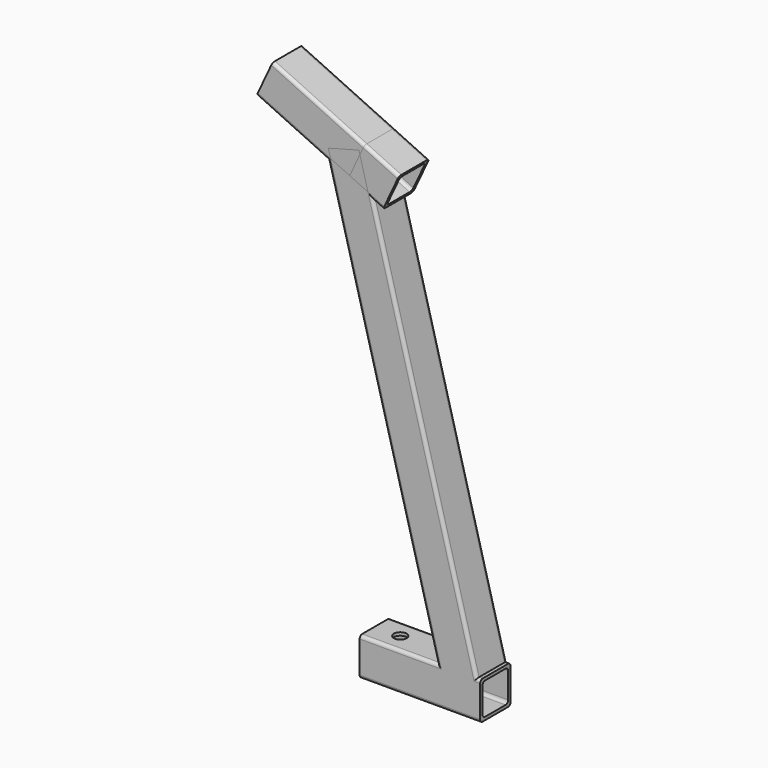
from build123d import *
from build123d import SkipClean  # not in build123d's __all__

# Parameters (mm, degrees)
F1_DEPTH       = 44.45
F1_DEPTH_BACK  = 76.2
F5_DEPTH       = 419.1
F5_DEPTH_BACK  = 28.956
F7_DEPTH       = 145.288
F10_DEPTH      = 38.1
F10_DEPTH_BACK = 101.6
F12_DEPTH      = 154.2941466414
F13_R          = 6.35
F14_DEPTH      = 6.35
F15_R          = 6.35
F16_DEPTH      = 6.35


with BuildPart() as f1:
    # F0 (on Right) → F1 (new body, two sides)
    with BuildSketch(Plane.YZ) as f1_sk:
        with BuildLine():
            ThreePointArc((19.05, 15.875), (18.1200640303, 18.1200640303), (15.875, 19.05))
            Line((15.875, 19.05), (-15.875, 19.05))
            ThreePointArc((-15.875, 19.05), (-18.1200640303, 18.1200640303), (-19.05, 15.875))
            Line((-19.05, 15.875), (-19.05, -15.875))
            ThreePointArc((-19.05, -15.875), (-18.1200640303, -18.1200640303), (-15.875, -19.05))
            Line((-15.875, -19.05), (15.875, -19.05))
            ThreePointArc((15.875, -19.05), (18.1200640303, -18.1200640303), (19.05, -15.875))
            Line((19.05, -15.875), (19.05, 15.875))
        make_face()
        with BuildLine():
            Line((-16.002, -12.827), (-16.002, 12.827))
            ThreePointArc((-16.002, 12.827), (-15.0720640303, 15.0720640303), (-12.827, 16.002))
            Line((-12.827, 16.002), (12.827, 16.002))
            ThreePointArc((12.827, 16.002), (15.0720640303, 15.0720640303), (16.002, 12.827))
            Line((16.002, 12.827), (16.002, -12.827))
            ThreePointArc((16.002, -12.827), (15.0720640303, -15.0720640303), (12.827, -16.002))
            Line((12.827, -16.002), (-12.827, -16.002))
            ThreePointArc((-12.827, -16.002), (-15.0720640303, -15.0720640303), (-16.002, -12.827))
        make_face(mode=Mode.SUBTRACT)
    extrude(amount=F1_DEPTH)
    extrude(f1_sk.sketch, amount=-F1_DEPTH_BACK)

    # F4 (on face) → F5 (join, two sides)
    with BuildSketch(Plane(origin=(-8.3589183447, 0, 31.1959079588), x_dir=(0.9659258263, 0, 0.2588190451), z_dir=(0.2588190451, 0, -0.9659258263))) as f5_sk:
        with BuildLine():
            ThreePointArc((44.45, 15.875), (43.5200640303, 18.1200640303), (41.275, 19.05))
            Line((41.275, 19.05), (9.525, 19.05))
            ThreePointArc((9.525, 19.05), (7.2799359697, 18.1200640303), (6.35, 15.875))
            Line((6.35, 15.875), (6.35, -15.875))
            ThreePointArc((6.35, -15.875), (7.2799359697, -18.1200640303), (9.525, -19.05))
            Line((9.525, -19.05), (41.275, -19.05))
            ThreePointArc((41.275, -19.05), (43.5200640303, -18.1200640303), (44.45, -15.875))
            Line((44.45, -15.875), (44.45, 15.875))
        make_face()
        with BuildLine():
            Line((12.573, 16.002), (38.227, 16.002))
            ThreePointArc((38.227, 16.002), (40.4720640303, 15.0720640303), (41.402, 12.827))
            Line((41.402, 12.827), (41.402, -12.827))
            ThreePointArc((41.402, -12.827), (40.4720640303, -15.0720640303), (38.227, -16.002))
            Line((38.227, -16.002), (12.573, -16.002))
            ThreePointArc((12.573, -16.002), (10.3279359697, -15.0720640303), (9.398, -12.827))
            Line((9.398, -12.827), (9.398, 12.827))
            ThreePointArc((9.398, 12.827), (10.3279359697, 15.0720640303), (12.573, 16.002))
        make_face(mode=Mode.SUBTRACT)
    extrude(amount=-F5_DEPTH)
    extrude(f5_sk.sketch, amount=F5_DEPTH_BACK)

    # F6 (on face) → F7 (cut)
    with BuildSketch(Plane(origin=(-76.2, 0, 0), x_dir=(0, -1, 0), z_dir=(-1, 0, 0))):
        with BuildLine():
            Line((12.827, 16.002), (-12.827, 16.002))
            ThreePointArc((-12.827, 16.002), (-15.0720640303, 15.0720640303), (-16.002, 12.827))
            Line((-16.002, 12.827), (-16.002, -12.827))
            ThreePointArc((-16.002, -12.827), (-15.0720640303, -15.0720640303), (-12.827, -16.002))
            Line((-12.827, -16.002), (12.827, -16.002))
            ThreePointArc((12.827, -16.002), (15.0720640303, -15.0720640303), (16.002, -12.827))
            Line((16.002, -12.827), (16.002, 12.827))
            ThreePointArc((16.002, 12.827), (15.0720640303, 15.0720640303), (12.827, 16.002))
        make_face()
    with SkipClean():  # cleaning this boolean's faces spoils the solid; the shape is the same uncleaned
        extrude(amount=-F7_DEPTH, mode=Mode.SUBTRACT)

    # F9 (on face) → F10 (join, two sides)
    with BuildSketch(Plane(origin=(-232.1066250318, 0, 108.2330967608), x_dir=(0, 1, 0), z_dir=(0.906307787, 0, -0.4226182617))) as f10_sk:
        with BuildLine():
            ThreePointArc((19.05, 377.0523048448), (18.1200640303, 379.297368875), (15.875, 380.2273048448))
            Line((15.875, 380.2273048448), (-15.875, 380.2273048448))
            ThreePointArc((-15.875, 380.2273048448), (-18.1200640303, 379.297368875), (-19.05, 377.0523048448))
            Line((-19.05, 377.0523048448), (-19.05, 345.3023048448))
            ThreePointArc((-19.05, 345.3023048448), (-18.1200640303, 343.0572408145), (-15.875, 342.1273048448))
            Line((-15.875, 342.1273048448), (15.875, 342.1273048448))
            ThreePointArc((15.875, 342.1273048448), (18.1200640303, 343.0572408145), (19.05, 345.3023048448))
            Line((19.05, 345.3023048448), (19.05, 377.0523048448))
        make_face()
        with BuildLine():
            Line((-12.827, 377.1793048448), (12.827, 377.1793048448))
            ThreePointArc((12.827, 377.1793048448), (15.0720640303, 376.249368875), (16.002, 374.0043048448))
            Line((16.002, 374.0043048448), (16.002, 348.3503048448))
            ThreePointArc((16.002, 348.3503048448), (15.0720640303, 346.1052408145), (12.827, 345.1753048448))
            Line((12.827, 345.1753048448), (-12.827, 345.1753048448))
            ThreePointArc((-12.827, 345.1753048448), (-15.0720640303, 346.1052408145), (-16.002, 348.3503048448))
            Line((-16.002, 348.3503048448), (-16.002, 374.0043048448))
            ThreePointArc((-16.002, 374.0043048448), (-15.0720640303, 376.249368875), (-12.827, 377.1793048448))
        make_face(mode=Mode.SUBTRACT)
    with SkipClean():  # cleaning this boolean's faces spoils the solid; the shape is the same uncleaned
        extrude(amount=F10_DEPTH)
        extrude(f10_sk.sketch, amount=-F10_DEPTH_BACK)

    # F11 (on face) → F12 (cut, through all)
    with BuildSketch(Plane(origin=(-197.5762983457, 0, 92.1313409885), x_dir=(0, 1, 0), z_dir=(0.906307787, 0, -0.4226182617))):
        with BuildLine():
            ThreePointArc((-12.827, 377.1793048448), (-15.0720640303, 376.249368875), (-16.002, 374.0043048448))
            Line((-16.002, 374.0043048448), (-16.002, 348.3503048448))
            ThreePointArc((-16.002, 348.3503048448), (-15.0720640303, 346.1052408145), (-12.827, 345.1753048448))
            Line((-12.827, 345.1753048448), (12.827, 345.1753048448))
            ThreePointArc((12.827, 345.1753048448), (15.0720640303, 346.1052408145), (16.002, 348.3503048448))
            Line((16.002, 348.3503048448), (16.002, 374.0043048448))
            ThreePointArc((16.002, 374.0043048448), (15.0720640303, 376.249368875), (12.827, 377.1793048448))
            Line((12.827, 377.1793048448), (-12.827, 377.1793048448))
        make_face()
    with SkipClean():  # cleaning this boolean's faces spoils the solid; the shape is the same uncleaned
        extrude(amount=-F12_DEPTH, mode=Mode.SUBTRACT)

    # F13 (on face) → F14 (cut)
    with BuildSketch(Plane.XY.offset(19.05)):
        with Locations((-50.8, 0)):
            Circle(F13_R)
    with SkipClean():  # cleaning this boolean's faces spoils the solid; the shape is the same uncleaned
        extrude(amount=-F14_DEPTH, mode=Mode.SUBTRACT)

    # F15 (on face) → F16 (cut)
    with BuildSketch(Plane(origin=(144.5892468675, 0, 310.0726405387), x_dir=(0.906307787, 0, -0.4226182617), z_dir=(-0.4226182617, 0, -0.906307787))):
        with Locations((-332.301324905, 0)):
            Circle(F15_R)
    with SkipClean():  # cleaning this boolean's faces spoils the solid; the shape is the same uncleaned
        extrude(amount=-F16_DEPTH, mode=Mode.SUBTRACT)


solid = f1.part
